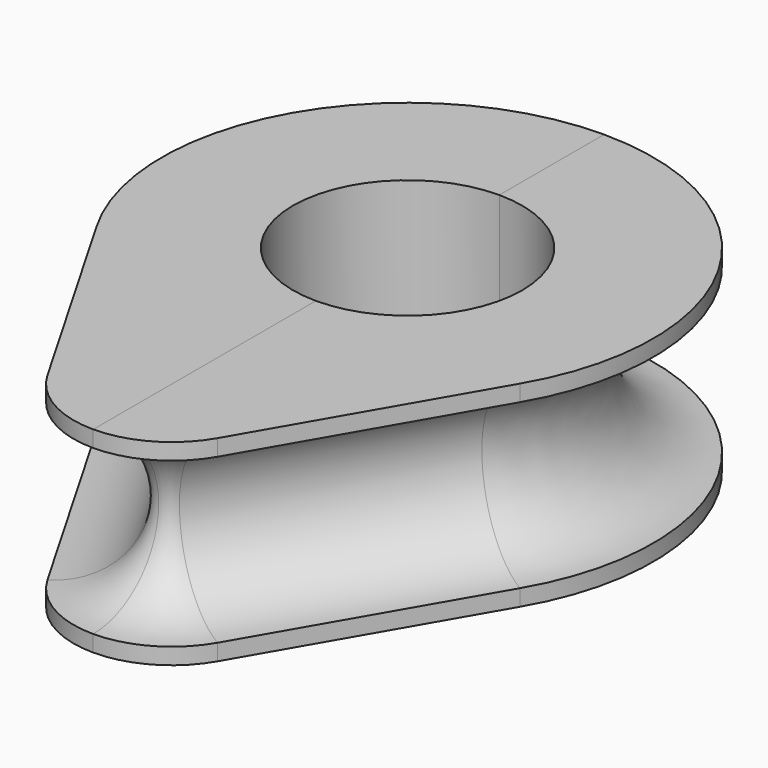
from build123d import *
from build123d import SkipClean  # not in build123d's __all__

# Parameters (mm, degrees)
F1_DEPTH = 6
F9_DEPTH = 25


with BuildPart() as f1:
    # F0 (on Top) → F1 (new body)
    with BuildSketch(Plane.XY):
        with BuildLine():
            Line((0, 3.5), (0, 7.5))
            ThreePointArc((0, 7.5), (-6.5081460588, 3.7274703054), (-6.4690456472, -3.7949240327))
            Line((-6.4690456472, -3.7949240327), (-2.5980762114, -10.4996397702))
            ThreePointArc((-2.5980762114, -10.4996397702), (-1.5, -11.5977159815), (0, -11.9996397702))
            Line((0, -11.9996397702), (0, -3.5))
            ThreePointArc((0, -3.5), (-3.5, 0), (0, 3.5))
        make_face()
    extrude(amount=F1_DEPTH)

    # F4: sweep along a path in F4_path
    with BuildLine(Plane(origin=(-2.5980762114, -10.4996397702, 0), x_dir=(0.5, -0.8660254038, 0), z_dir=(0.8660254038, 0.5, 0))) as f4_path:
        Line((0, 0), (-7.7419388717, 0))
    # F3 (on face) → F4 (sweep, cut)
    with BuildSketch(Plane(origin=(3.8969583329, -6.7497298276, 0), x_dir=(0.8660254038, 0.5, 0), z_dir=(0.5, -0.8660254038, 0))):
        with BuildLine():
            ThreePointArc((-7.4998198851, 0.5), (-4.9998198851, 3), (-7.4998198851, 5.5))
            Line((-7.4998198851, 5.5), (-7.4998198851, 0.5))
        make_face()
    sweep(path=f4_path.line, mode=Mode.SUBTRACT)

    # F7: sweep along a path in F0
    with BuildLine(Plane.XY) as f7_path:
        ThreePointArc((0, 7.5), (-6.5081460588, 3.7274703054), (-6.4690456472, -3.7949240327))
    # F6 (on face) → F7 (sweep, cut)
    with BuildSketch(Plane(origin=(0.0259888971, -0.0450140902, 0), x_dir=(-0.8660254038, -0.5, 0), z_dir=(-0.5, 0.8660254038, 0))):
        with BuildLine():
            ThreePointArc((7.4998198851, 5.5), (4.9998198851, 3), (7.4998198851, 0.5))
            Line((7.4998198851, 0.5), (7.4998198851, 5.5))
        make_face()
    sweep(path=f7_path.line, mode=Mode.SUBTRACT)

    # F8 (on face) → F9 (cut)
    with BuildSketch(Plane.YZ):
        with BuildLine():
            Line((7.5, 0.5), (7.5, 5.5))
            add(Edge.make_bspline(
                [(7.5, 5.5), (5.0000600383, 5.5), (5.0000600383, 3), (5.0000600383, 0.5), (7.5, 0.5)],
                knots=[0, 0, 0, 1.5707963268, 1.5707963268, 3.1415926536, 3.1415926536, 3.1415926536], degree=2, weights=[1, 0.7071067812, 1, 0.7071067812, 1]))
        make_face()
    extrude(amount=-F9_DEPTH, mode=Mode.SUBTRACT)

    # F11: sweep along a path in F0
    with BuildLine(Plane.XY) as f11_path:
        ThreePointArc((-2.5980762114, -10.4996397702), (-1.5, -11.5977159815), (0, -11.9996397702))
    # F10 (on face) → F11 (sweep, cut)
    with BuildSketch(Plane(origin=(3.8969583329, -6.7497298276, 0), x_dir=(-0.8660254038, -0.5, 0), z_dir=(-0.5, 0.8660254038, 0))):
        with BuildLine():
            ThreePointArc((7.4998198851, 5.5), (4.9998198851, 3), (7.4998198851, 0.5))
            Line((7.4998198851, 0.5), (7.4998198851, 5.5))
        make_face()
    sweep(path=f11_path.line, mode=Mode.SUBTRACT)

    # F12: F1 across plane


with BuildPart() as f1_1:
    add(f1.part, clean=False)
    with SkipClean():  # cleaning this boolean's faces spoils the solid; the shape is the same uncleaned
        add(f1.part.mirror(Plane.YZ), clean=False)


solid = f1_1.part
